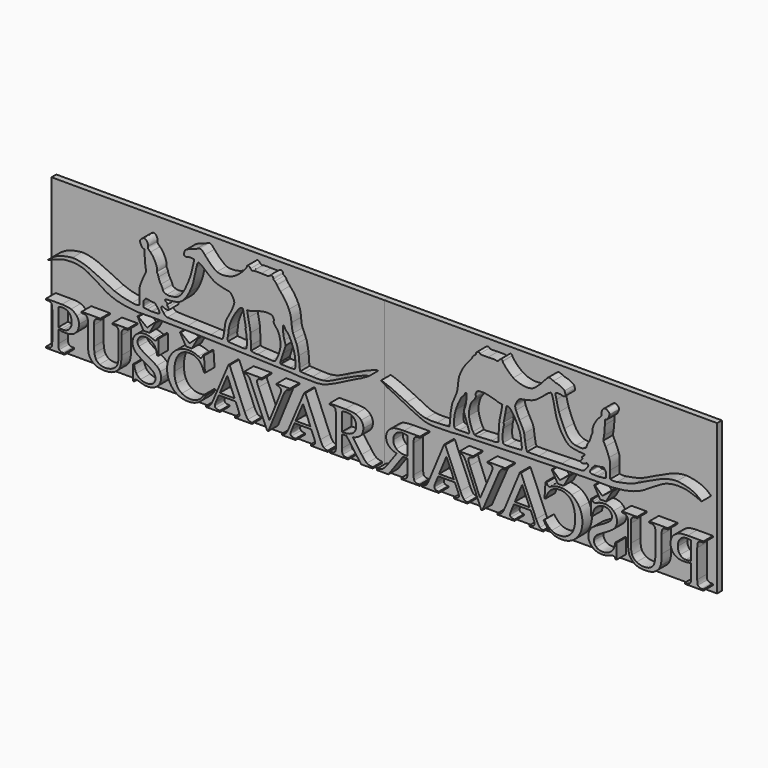
from build123d import *

# Parameters (mm, degrees)
F1_DEPTH = 2
F2_W     = 55.653892
F2_H     = 25.0897646814
F3_DEPTH = 1


# Not quite as in the source:
# - ends of sketch curves that miss each other by under 0.0002 mm in the source are joined


with BuildPart() as f1:
    # F0 (on Front) → F1 (new body)
    with BuildSketch(Plane.XZ):
        with BuildLine():
            add(Edge.make_bspline(
                [(14.906345, -1.877976), (14.32217, -1.779452), (13.148397, -1.722864), (11.136232, -1.696216)],
                knots=[0, 0, 0, 0, 1, 1, 1, 1], degree=3))
            add(Edge.make_bspline(
                [(17.93175, -1.917631), (17.120906, -1.922429), (15.472308, -1.914696), (14.906345, -1.877976)],
                knots=[0, 0, 0, 0, 1, 1, 1, 1], degree=3))
            add(Edge.make_bspline(
                [(21.221287, -0.880716), (18.995206, -1.990873), (18.702316, -1.788918), (17.93175, -1.917631)],
                knots=[0, 0, 0, 0, 1, 1, 1, 1], degree=3))
            add(Edge.make_bspline(
                [(24.850025, 0.960048), (24.039003, 0.584379), (23.127224, 0.069786), (21.221287, -0.880716)],
                knots=[0, 0, 0, 0, 1, 1, 1, 1], degree=3))
            add(Edge.make_bspline(
                [(26.655553, 1.91644), (25.579851, 1.29154), (25.170539, 1.055504), (24.850025, 0.960048)],
                knots=[0, 0, 0, 0, 1, 1, 1, 1], degree=3))
            add(Edge.make_bspline(
                [(22.267048, 0.156324), (24.465708, 1.272403), (26.336585, 2.022764), (26.655553, 1.91644)],
                knots=[0, 0, 0, 0, 1, 1, 1, 1], degree=3))
            add(Edge.make_bspline(
                [(19.081687, -1.170408), (19.8364, -1.054392), (20.090223, -0.948672), (22.267048, 0.156324)],
                knots=[0, 0, 0, 0, 1, 1, 1, 1], degree=3))
            add(Edge.make_bspline(
                [(17.243755, -1.222769), (17.960379, -1.274655), (18.504328, -1.259159), (19.081687, -1.170408)],
                knots=[0, 0, 0, 0, 1, 1, 1, 1], degree=3))
            add(Edge.make_bspline(
                [(15.753238, -1.157751), (16.121207, -1.200516), (16.683927, -1.182247), (17.243755, -1.222769)],
                knots=[0, 0, 0, 0, 1, 1, 1, 1], degree=3))
            Line((15.753238, -1.157751), (15.198408, -1.093263))
            Line((15.198408, -1.093263), (15.088607, -0.617193))
            add(Edge.make_bspline(
                [(14.94541, 1.125097), (15.075639, 0.479813), (15.009153, -0.272688), (15.088607, -0.617193)],
                knots=[0, 0, 0, 0, 1, 1, 1, 1], degree=3))
            add(Edge.make_bspline(
                [(14.582732, 2.719921), (14.739998, 2.461315), (14.74895, 2.098563), (14.94541, 1.125097)],
                knots=[0, 0, 0, 0, 1, 1, 1, 1], degree=3))
            add(Edge.make_bspline(
                [(14.328207, 3.347891), (14.44461, 3.112924), (14.481984, 2.885585), (14.582732, 2.719921)],
                knots=[0, 0, 0, 0, 1, 1, 1, 1], degree=3))
            add(Edge.make_bspline(
                [(13.999418, 4.123104), (14.095811, 3.931701), (14.222803, 3.560655), (14.328207, 3.347891)],
                knots=[0, 0, 0, 0, 1, 1, 1, 1], degree=3))
            add(Edge.make_bspline(
                [(13.727534, 5.573331), (13.790834, 4.851254), (13.884605, 4.351086), (13.999418, 4.123104)],
                knots=[0, 0, 0, 0, 1, 1, 1, 1], degree=3))
            add(Edge.make_bspline(
                [(13.308524, 7.419482), (13.576491, 6.801128), (13.647219, 6.489506), (13.727534, 5.573331)],
                knots=[0, 0, 0, 0, 1, 1, 1, 1], degree=3))
            add(Edge.make_bspline(
                [(11.873043, 9.590299), (12.525854, 8.877087), (12.963999, 8.214497), (13.308524, 7.419482)],
                knots=[0, 0, 0, 0, 1, 1, 1, 1], degree=3))
            add(Edge.make_bspline(
                [(11.312471, 10.358717), (11.397874, 10.179621), (11.650133, 9.833834), (11.873043, 9.590299)],
                knots=[0, 0, 0, 0, 1, 1, 1, 1], degree=3))
            add(Edge.make_bspline(
                [(10.93464, 10.785747), (11.057043, 10.729977), (11.227065, 10.537815), (11.312471, 10.358717)],
                knots=[0, 0, 0, 0, 1, 1, 1, 1], degree=3))
            add(Edge.make_bspline(
                [(10.712094, 11.058823), (10.712094, 10.964399), (10.81224, 10.841517), (10.93464, 10.785747)],
                knots=[0, 0, 0, 0, 1, 1, 1, 1], degree=3))
            add(Edge.make_bspline(
                [(10.041345, 11.302095), (10.278685, 11.588074), (10.712094, 11.430879), (10.712094, 11.058823)],
                knots=[0, 0, 0, 0, 1, 1, 1, 1], degree=3))
            add(Edge.make_bspline(
                [(8.698811, 11.201489), (9.752135, 11.154643), (9.930034, 11.167972), (10.041345, 11.302095)],
                knots=[0, 0, 0, 0, 1, 1, 1, 1], degree=3))
            add(Edge.make_bspline(
                [(7.316055, 11.150237), (7.429841, 11.221298), (7.879037, 11.237946), (8.698811, 11.201489)],
                knots=[0, 0, 0, 0, 1, 1, 1, 1], degree=3))
            add(Edge.make_bspline(
                [(6.894993, 11.345097), (7.105031, 11.09548), (7.175878, 11.062695), (7.316055, 11.150237)],
                knots=[0, 0, 0, 0, 1, 1, 1, 1], degree=3))
            add(Edge.make_bspline(
                [(6.253564, 11.386014), (6.324227, 11.736813), (6.579065, 11.720557), (6.894993, 11.345097)],
                knots=[0, 0, 0, 0, 1, 1, 1, 1], degree=3))
            add(Edge.make_bspline(
                [(4.478759, 9.532788), (5.163673, 9.984654), (6.186398, 11.052569), (6.253564, 11.386014)],
                knots=[0, 0, 0, 0, 1, 1, 1, 1], degree=3))
            add(Edge.make_bspline(
                [(1.271998, 9.038063), (2.051735, 8.694703), (3.561472, 8.927619), (4.478759, 9.532788)],
                knots=[0, 0, 0, 0, 1, 1, 1, 1], degree=3))
            add(Edge.make_bspline(
                [(-0.752399, 10.868156), (-0.091398, 10.050352), (0.796987, 9.247235), (1.271998, 9.038063)],
                knots=[0, 0, 0, 0, 1, 1, 1, 1], degree=3))
            add(Edge.make_bspline(
                [(-2.225738, 11.266098), (-1.473508, 11.658181), (-1.367889, 11.629654), (-0.752399, 10.868156)],
                knots=[0, 0, 0, 0, 1, 1, 1, 1], degree=3))
            add(Edge.make_bspline(
                [(-2.774897, 11.079693), (-2.669555, 11.079693), (-2.42243, 11.163575), (-2.225738, 11.266098)],
                knots=[0, 0, 0, 0, 1, 1, 1, 1], degree=3))
            add(Edge.make_bspline(
                [(-4.08105, 10.424963), (-3.987386, 10.604222), (-3.038848, 11.079693), (-2.774897, 11.079693)],
                knots=[0, 0, 0, 0, 1, 1, 1, 1], degree=3))
            add(Edge.make_bspline(
                [(-4.219618, 9.989076), (-4.185483, 10.148283), (-4.123126, 10.344431), (-4.08105, 10.424963)],
                knots=[0, 0, 0, 0, 1, 1, 1, 1], degree=3))
            add(Edge.make_bspline(
                [(-4.061568, 9.599316), (-4.246722, 9.683681), (-4.271826, 9.745583), (-4.219618, 9.989076)],
                knots=[0, 0, 0, 0, 1, 1, 1, 1], degree=3))
            add(Edge.make_bspline(
                [(-3.610077, 9.613738), (-3.778781, 9.530104), (-3.901071, 9.526198), (-4.061568, 9.599316)],
                knots=[0, 0, 0, 0, 1, 1, 1, 1], degree=3))
            add(Edge.make_bspline(
                [(-2.931005, 9.687685), (-3.179434, 9.710291), (-3.481691, 9.677384), (-3.610077, 9.613738)],
                knots=[0, 0, 0, 0, 1, 1, 1, 1], degree=3))
            add(Edge.make_bspline(
                [(-2.725248, 8.702524), (-2.519345, 9.684477), (-2.413054, 9.640532), (-2.931005, 9.687685)],
                knots=[0, 0, 0, 0, 1, 1, 1, 1], degree=3))
            add(Edge.make_bspline(
                [(-3.15726, 6.987366), (-2.958632, 7.561011), (-2.79805, 8.355337), (-2.725248, 8.702524)],
                knots=[0, 0, 0, 0, 1, 1, 1, 1], degree=3))
            add(Edge.make_bspline(
                [(-4.059426, 4.808949), (-3.614686, 5.727312), (-3.417731, 6.235111), (-3.15726, 6.987366)],
                knots=[0, 0, 0, 0, 1, 1, 1, 1], degree=3))
            add(Edge.make_bspline(
                [(-6.004577, 2.986056), (-5.607307, 3.019452), (-4.839203, 3.198762), (-4.059426, 4.808949)],
                knots=[0, 0, 0, 0, 1, 1, 1, 1], degree=3))
            add(Edge.make_bspline(
                [(-7.133794, 2.942523), (-6.823922, 2.823849), (-6.26808, 2.963916), (-6.004577, 2.986056)],
                knots=[0, 0, 0, 0, 1, 1, 1, 1], degree=3))
            add(Edge.make_bspline(
                [(-7.76966, 3.423622), (-7.718225, 3.172137), (-7.620435, 3.128897), (-7.133794, 2.942523)],
                knots=[0, 0, 0, 0, 1, 1, 1, 1], degree=3))
            add(Edge.make_bspline(
                [(-8.10803, 4.135725), (-7.954679, 3.904204), (-7.802412, 3.583758), (-7.76966, 3.423622)],
                knots=[0, 0, 0, 0, 1, 1, 1, 1], degree=3))
            add(Edge.make_bspline(
                [(-8.505055, 5.084853), (-8.440045, 4.79435), (-8.261384, 4.367243), (-8.10803, 4.135725)],
                knots=[0, 0, 0, 0, 1, 1, 1, 1], degree=3))
            add(Edge.make_bspline(
                [(-8.717103, 5.613037), (-8.665487, 5.613037), (-8.570068, 5.375352), (-8.505055, 5.084853)],
                knots=[0, 0, 0, 0, 1, 1, 1, 1], degree=3))
            add(Edge.make_bspline(
                [(-8.753904, 5.792768), (-8.785276, 5.693914), (-8.768721, 5.613037), (-8.717103, 5.613037)],
                knots=[0, 0, 0, 0, 1, 1, 1, 1], degree=3))
            add(Edge.make_bspline(
                [(-9.860368, 8.304478), (-9.203417, 7.699323), (-8.59043, 6.307826), (-8.753904, 5.792768)],
                knots=[0, 0, 0, 0, 1, 1, 1, 1], degree=3))
            add(Edge.make_bspline(
                [(-10.277738, 8.987698), (-10.318358, 8.775202), (-10.250137, 8.663509), (-9.860368, 8.304478)],
                knots=[0, 0, 0, 0, 1, 1, 1, 1], degree=3))
            add(Edge.make_bspline(
                [(-11.029922, 9.981411), (-10.634264, 10.121534), (-10.176578, 9.516885), (-10.277738, 8.987698)],
                knots=[0, 0, 0, 0, 1, 1, 1, 1], degree=3))
            add(Edge.make_bspline(
                [(-11.625832, 9.412821), (-11.625832, 9.560629), (-11.276268, 9.894165), (-11.029922, 9.981411)],
                knots=[0, 0, 0, 0, 1, 1, 1, 1], degree=3))
            add(Edge.make_bspline(
                [(-11.426944, 8.863732), (-11.536331, 9.096444), (-11.625832, 9.343532), (-11.625832, 9.412821)],
                knots=[0, 0, 0, 0, 1, 1, 1, 1], degree=3))
            add(Edge.make_bspline(
                [(-11.017363, 8.440622), (-11.174629, 8.440622), (-11.278492, 8.547917), (-11.426944, 8.863732)],
                knots=[0, 0, 0, 0, 1, 1, 1, 1], degree=3))
            add(Edge.make_bspline(
                [(-10.814299, 7.568784), (-10.806933, 8.410669), (-10.814017, 8.440622), (-11.017363, 8.440622)],
                knots=[0, 0, 0, 0, 1, 1, 1, 1], degree=3))
            add(Edge.make_bspline(
                [(-10.689455, 5.941008), (-10.762316, 6.356772), (-10.818496, 7.089271), (-10.814299, 7.568784)],
                knots=[0, 0, 0, 0, 1, 1, 1, 1], degree=3))
            Line((-10.689455, 5.941008), (-10.556977, 5.185073))
            Line((-10.556977, 5.185073), (-10.933549, 4.432964))
            add(Edge.make_bspline(
                [(-11.528657, 3.000977), (-11.408461, 3.374908), (-11.140663, 4.019303), (-10.933549, 4.432964)],
                knots=[0, 0, 0, 0, 1, 1, 1, 1], degree=3))
            add(Edge.make_bspline(
                [(-11.680447, 1.180009), (-11.741371, 2.221567), (-11.728129, 2.380402), (-11.528657, 3.000977)],
                knots=[0, 0, 0, 0, 1, 1, 1, 1], degree=3))
            add(Edge.make_bspline(
                [(-11.725561, -0.095861), (-11.644368, 0.001968), (-11.632001, 0.351755), (-11.680447, 1.180009)],
                knots=[0, 0, 0, 0, 1, 1, 1, 1], degree=3))
            add(Edge.make_bspline(
                [(-12.910174, -0.133882), (-12.705955, -0.185907), (-11.856695, -0.253869), (-11.725561, -0.095861)],
                knots=[0, 0, 0, 0, 1, 1, 1, 1], degree=3))
            add(Edge.make_bspline(
                [(-15.904108, 0.64861), (-14.299201, 0.005744), (-13.8899, 0.095759), (-12.910174, -0.133882)],
                knots=[0, 0, 0, 0, 1, 1, 1, 1], degree=3))
            add(Edge.make_bspline(
                [(-22.904303, 3.242929), (-20.452492, 3.2672), (-17.509014, 1.291476), (-15.904108, 0.64861)],
                knots=[0, 0, 0, 0, 1, 1, 1, 1], degree=3))
            add(Edge.make_bspline(
                [(-26.998339, 1.579359), (-25.865313, 2.728317), (-24.513767, 3.060715), (-22.904303, 3.242929)],
                knots=[0, 0, 0, 0, 1, 1, 1, 1], degree=3))
            add(Edge.make_bspline(
                [(-22.929805, 2.60097), (-24.746773, 2.592249), (-25.035387, 2.340363), (-26.998339, 1.579359)],
                knots=[0, 0, 0, 0, 1, 1, 1, 1], degree=3))
            add(Edge.make_bspline(
                [(-17.952161, 0.517718), (-20.188597, 1.791212), (-20.672504, 2.477729), (-22.929805, 2.60097)],
                knots=[0, 0, 0, 0, 1, 1, 1, 1], degree=3))
            add(Edge.make_bspline(
                [(-9.194343, -1.180633), (-13.817713, -1.465037), (-16.547222, -0.573734), (-17.952161, 0.517718)],
                knots=[0, 0, 0, 0, 1, 1, 1, 1], degree=3))
            add(Edge.make_bspline(
                [(-3.162159, -1.26493), (-3.716969, -1.21299), (-6.431622, -1.212044), (-9.194343, -1.180633)],
                knots=[0, 0, 0, 0, 1, 1, 1, 1], degree=3))
            add(Edge.make_bspline(
                [(1.993705, -1.411014), (-0.287212, -1.382608), (-2.607353, -1.31687), (-3.162159, -1.26493)],
                knots=[0, 0, 0, 0, 1, 1, 1, 1], degree=3))
            add(Edge.make_bspline(
                [(7.177613, -1.560089), (6.607383, -1.506504), (4.274625, -1.43942), (1.993705, -1.411014)],
                knots=[0, 0, 0, 0, 1, 1, 1, 1], degree=3))
            add(Edge.make_bspline(
                [(11.136232, -1.696216), (9.529222, -1.674937), (7.747843, -1.613678), (7.177613, -1.560089)],
                knots=[0, 0, 0, 0, 1, 1, 1, 1], degree=3))
        make_face()
        with BuildLine():
            add(Edge.make_bspline(
                [(-8.910165, -0.345128), (-8.490871, -0.342588), (-8.182475, -0.281318), (-8.373864, 0.074051)],
                knots=[0, 0, 0, 0, 1, 1, 1, 1], degree=3))
            add(Edge.make_bspline(
                [(-9.495381, -0.358754), (-9.387612, -0.349412), (-9.289241, -0.364709), (-8.910165, -0.345128)],
                knots=[0, 0, 0, 0, 1, 1, 1, 1], degree=3))
            add(Edge.make_bspline(
                [(-9.738335, -0.368462), (-9.638846, -0.372809), (-9.59257, -0.361435), (-9.495381, -0.358754)],
                knots=[0, 0, 0, 0, 1, 1, 1, 1], degree=3))
            add(Edge.make_bspline(
                [(-10.404219, -0.294599), (-10.152152, -0.315992), (-9.923366, -0.360371), (-9.738335, -0.368462)],
                knots=[0, 0, 0, 0, 1, 1, 1, 1], degree=3))
            add(Edge.make_bspline(
                [(-10.839261, -0.242123), (-10.691761, -0.281312), (-10.522207, -0.284589), (-10.404219, -0.294599)],
                knots=[0, 0, 0, 0, 1, 1, 1, 1], degree=3))
            add(Edge.make_bspline(
                [(-11.026996, 0.280505), (-11.000777, -0.125859), (-11.080697, -0.177971), (-10.839261, -0.242123)],
                knots=[0, 0, 0, 0, 1, 1, 1, 1], degree=3))
            add(Edge.make_bspline(
                [(-10.914375, 0.886837), (-10.999324, 0.787582), (-11.045656, 0.569619), (-11.026996, 0.280505)],
                knots=[0, 0, 0, 0, 1, 1, 1, 1], degree=3))
            add(Edge.make_bspline(
                [(-10.715185, 1.149182), (-10.746774, 1.059983), (-10.841429, 0.972062), (-10.914375, 0.886837)],
                knots=[0, 0, 0, 0, 1, 1, 1, 1], degree=3))
            add(Edge.make_bspline(
                [(-10.392712, 1.227538), (-10.479397, 1.236061), (-10.662466, 1.298051), (-10.715185, 1.149182)],
                knots=[0, 0, 0, 0, 1, 1, 1, 1], degree=3))
            add(Edge.make_bspline(
                [(-9.543734, 1.088922), (-9.794588, 1.088922), (-10.164671, 1.205107), (-10.392712, 1.227538)],
                knots=[0, 0, 0, 0, 1, 1, 1, 1], degree=3))
            add(Edge.make_bspline(
                [(-8.986752, 0.900417), (-9.066299, 1.049052), (-9.184099, 1.088922), (-9.543734, 1.088922)],
                knots=[0, 0, 0, 0, 1, 1, 1, 1], degree=3))
            add(Edge.make_bspline(
                [(-8.78139, 0.684514), (-8.911655, 0.723077), (-8.927756, 0.790184), (-8.986752, 0.900417)],
                knots=[0, 0, 0, 0, 1, 1, 1, 1], degree=3))
            add(Edge.make_bspline(
                [(-8.607045, 0.434798), (-8.682339, 0.537321), (-8.674041, 0.652736), (-8.78139, 0.684514)],
                knots=[0, 0, 0, 0, 1, 1, 1, 1], degree=3))
            add(Edge.make_bspline(
                [(-8.373864, 0.074051), (-8.403811, 0.147174), (-8.50376, 0.294159), (-8.607045, 0.434798)],
                knots=[0, 0, 0, 0, 1, 1, 1, 1], degree=3))
        make_face(mode=Mode.SUBTRACT)
        with BuildLine():
            add(Edge.make_bspline(
                [(-7.048802, 1.502837), (-7.127644, 1.407839), (-6.992671, 1.331672), (-6.912331, 1.181793)],
                knots=[0, 0, 0, 0, 1, 1, 1, 1], degree=3))
            add(Edge.make_bspline(
                [(-7.01613, 2.215528), (-8.157323, 2.174605), (-6.659226, 1.665838), (-7.048802, 1.502837)],
                knots=[0, 0, 0, 0, 1, 1, 1, 1], degree=3))
            add(Edge.make_bspline(
                [(-5.578315, 2.386771), (-5.898216, 2.288126), (-6.814231, 2.205943), (-7.01613, 2.215528)],
                knots=[0, 0, 0, 0, 1, 1, 1, 1], degree=3))
            add(Edge.make_bspline(
                [(-4.531857, 2.871073), (-4.817808, 2.612456), (-5.229875, 2.43191), (-5.578315, 2.386771)],
                knots=[0, 0, 0, 0, 1, 1, 1, 1], degree=3))
            add(Edge.make_bspline(
                [(-3.354824, 4.508436), (-3.671204, 3.862607), (-4.280098, 3.049649), (-4.531857, 2.871073)],
                knots=[0, 0, 0, 0, 1, 1, 1, 1], degree=3))
            add(Edge.make_bspline(
                [(-2.175694, 8.560992), (-2.56428, 6.342971), (-2.855096, 5.528526), (-3.354824, 4.508436)],
                knots=[0, 0, 0, 0, 1, 1, 1, 1], degree=3))
            add(Edge.make_bspline(
                [(-1.750597, 9.378886), (-1.916109, 9.383035), (-1.998193, 9.290254), (-2.175694, 8.560992)],
                knots=[0, 0, 0, 0, 1, 1, 1, 1], degree=3))
            add(Edge.make_bspline(
                [(-1.01849, 8.928364), (-1.281574, 9.170691), (-1.530667, 9.303115), (-1.750597, 9.378886)],
                knots=[0, 0, 0, 0, 1, 1, 1, 1], degree=3))
            add(Edge.make_bspline(
                [(1.060771, 7.356657), (0.581654, 7.56871), (-0.109819, 8.091391), (-1.01849, 8.928364)],
                knots=[0, 0, 0, 0, 1, 1, 1, 1], degree=3))
            add(Edge.make_bspline(
                [(3.218205, 6.838342), (2.839519, 6.838342), (1.510394, 7.157659), (1.060771, 7.356657)],
                knots=[0, 0, 0, 0, 1, 1, 1, 1], degree=3))
            add(Edge.make_bspline(
                [(4.060283, 5.880124), (3.873068, 6.370341), (3.461791, 6.838342), (3.218205, 6.838342)],
                knots=[0, 0, 0, 0, 1, 1, 1, 1], degree=3))
            add(Edge.make_bspline(
                [(4.033076, 4.899018), (4.214246, 5.435282), (4.215321, 5.474133), (4.060283, 5.880124)],
                knots=[0, 0, 0, 0, 1, 1, 1, 1], degree=3))
            add(Edge.make_bspline(
                [(3.448512, 3.633745), (3.666272, 4.02254), (3.929329, 4.591912), (4.033076, 4.899018)],
                knots=[0, 0, 0, 0, 1, 1, 1, 1], degree=3))
            add(Edge.make_bspline(
                [(2.663192, 1.913468), (2.757802, 2.28428), (2.756721, 2.398614), (3.448512, 3.633745)],
                knots=[0, 0, 0, 0, 1, 1, 1, 1], degree=3))
            add(Edge.make_bspline(
                [(2.512378, 0.792608), (2.600587, 1.204351), (2.582412, 1.596865), (2.663192, 1.913468)],
                knots=[0, 0, 0, 0, 1, 1, 1, 1], degree=3))
            add(Edge.make_bspline(
                [(2.327497, -0.227682), (2.400339, -0.041381), (2.435526, 0.43387), (2.512378, 0.792608)],
                knots=[0, 0, 0, 0, 1, 1, 1, 1], degree=3))
            Line((2.327497, -0.227682), (2.181902, -0.600062))
            add(Edge.make_bspline(
                [(0.232009, -0.576553), (0.872563, -0.617182), (1.590502, -0.61016), (2.181902, -0.600062)],
                knots=[0, 0, 0, 0, 1, 1, 1, 1], degree=3))
            add(Edge.make_bspline(
                [(-3.590776, -0.472679), (-2.393361, -0.51865), (-0.800696, -0.520315), (0.232009, -0.576553)],
                knots=[0, 0, 0, 0, 1, 1, 1, 1], degree=3))
            add(Edge.make_bspline(
                [(-7.041067, -0.368403), (-6.859287, -0.402507), (-5.306659, -0.449429), (-3.590776, -0.472679)],
                knots=[0, 0, 0, 0, 1, 1, 1, 1], degree=3))
            add(Edge.make_bspline(
                [(-7.632221, 0.08488), (-7.435851, -0.209899), (-7.290057, -0.321693), (-7.041067, -0.368403)],
                knots=[0, 0, 0, 0, 1, 1, 1, 1], degree=3))
            add(Edge.make_bspline(
                [(-8.025351, 0.604434), (-7.940803, 0.419496), (-7.781937, 0.282607), (-7.632221, 0.08488)],
                knots=[0, 0, 0, 0, 1, 1, 1, 1], degree=3))
            add(Edge.make_bspline(
                [(-8.01615, 0.874371), (-8.063264, 0.771642), (-8.052681, 0.682654), (-8.025351, 0.604434)],
                knots=[0, 0, 0, 0, 1, 1, 1, 1], degree=3))
            add(Edge.make_bspline(
                [(-7.581759, 0.873524), (-7.839657, 1.025868), (-7.864676, 1.025919), (-8.01615, 0.874371)],
                knots=[0, 0, 0, 0, 1, 1, 1, 1], degree=3))
            add(Edge.make_bspline(
                [(-6.912331, 1.181793), (-6.43918, 0.721799), (-7.058514, 0.564434), (-7.581759, 0.873524)],
                knots=[0, 0, 0, 0, 1, 1, 1, 1], degree=3))
        make_face(mode=Mode.SUBTRACT)
        with BuildLine():
            add(Edge.make_bspline(
                [(6.184643, -0.613849), (6.328788, -0.34451), (6.305863, 1.196601), (6.152122, 1.572216)],
                knots=[0, 0, 0, 0, 1, 1, 1, 1], degree=3))
            add(Edge.make_bspline(
                [(5.501306, -0.781379), (5.992971, -0.793769), (6.102745, -0.766873), (6.184643, -0.613849)],
                knots=[0, 0, 0, 0, 1, 1, 1, 1], degree=3))
            add(Edge.make_bspline(
                [(3.121473, -0.611176), (3.164935, -0.656425), (4.563654, -0.757717), (5.501306, -0.781379)],
                knots=[0, 0, 0, 0, 1, 1, 1, 1], degree=3))
            add(Edge.make_bspline(
                [(3.08674, 0.094678), (3.016108, -0.268195), (3.099525, -0.588342), (3.121473, -0.611176)],
                knots=[0, 0, 0, 0, 1, 1, 1, 1], degree=3))
            add(Edge.make_bspline(
                [(3.223189, 1.063934), (3.221213, 0.891205), (3.157369, 0.457551), (3.08674, 0.094678)],
                knots=[0, 0, 0, 0, 1, 1, 1, 1], degree=3))
            add(Edge.make_bspline(
                [(4.238692, 3.760612), (3.644372, 2.802936), (3.229257, 1.613852), (3.223189, 1.063934)],
                knots=[0, 0, 0, 0, 1, 1, 1, 1], degree=3))
            add(Edge.make_bspline(
                [(5.440293, 5.04752), (5.14241, 5.04752), (4.829064, 4.71193), (4.238692, 3.760612)],
                knots=[0, 0, 0, 0, 1, 1, 1, 1], degree=3))
            add(Edge.make_bspline(
                [(5.860931, 3.680854), (5.668032, 4.980261), (5.647328, 5.04752), (5.440293, 5.04752)],
                knots=[0, 0, 0, 0, 1, 1, 1, 1], degree=3))
            add(Edge.make_bspline(
                [(6.088227, 2.470529), (6.070475, 2.563722), (5.945584, 3.110624), (5.860931, 3.680854)],
                knots=[0, 0, 0, 0, 1, 1, 1, 1], degree=3))
            add(Edge.make_bspline(
                [(6.065339, 2.218417), (6.111804, 2.37303), (6.105979, 2.377334), (6.088227, 2.470529)],
                knots=[0, 0, 0, 0, 1, 1, 1, 1], degree=3))
            add(Edge.make_bspline(
                [(6.152122, 1.572216), (6.02902, 2.126563), (6.0532, 2.178031), (6.065339, 2.218417)],
                knots=[0, 0, 0, 0, 1, 1, 1, 1], degree=3))
        make_face(mode=Mode.SUBTRACT)
        with BuildLine():
            add(Edge.make_bspline(
                [(10.972119, -0.970234), (11.068069, -0.868905), (11.124229, -0.728688), (11.217681, -0.588627)],
                knots=[0, 0, 0, 0, 1, 1, 1, 1], degree=3))
            add(Edge.make_bspline(
                [(10.441141, -1.02308), (10.61234, -1.048169), (10.813135, -1.018564), (10.972119, -0.970234)],
                knots=[0, 0, 0, 0, 1, 1, 1, 1], degree=3))
            add(Edge.make_bspline(
                [(8.089973, -0.896675), (9.030035, -0.891257), (10.360984, -1.011331), (10.441141, -1.02308)],
                knots=[0, 0, 0, 0, 1, 1, 1, 1], degree=3))
            add(Edge.make_bspline(
                [(7.32374, -0.854751), (7.497097, -0.911963), (7.710503, -0.898868), (8.089973, -0.896675)],
                knots=[0, 0, 0, 0, 1, 1, 1, 1], degree=3))
            Line((7.32374, -0.854751), (6.95689, -0.750727))
            Line((6.95689, -0.750727), (6.977267, 0.080327))
            add(Edge.make_bspline(
                [(6.849149, 1.838394), (6.842037, 1.268164), (6.987723, 0.506474), (6.977267, 0.080327)],
                knots=[0, 0, 0, 0, 1, 1, 1, 1], degree=3))
            add(Edge.make_bspline(
                [(6.496809, 3.963612), (6.615602, 3.295945), (6.857469, 2.506058), (6.849149, 1.838394)],
                knots=[0, 0, 0, 0, 1, 1, 1, 1], degree=3))
            add(Edge.make_bspline(
                [(6.32084, 5.013676), (6.316155, 5.006367), (6.395353, 4.533842), (6.496809, 3.963612)],
                knots=[0, 0, 0, 0, 1, 1, 1, 1], degree=3))
            add(Edge.make_bspline(
                [(6.708351, 5.069511), (6.499893, 5.046115), (6.325514, 5.02098), (6.32084, 5.013676)],
                knots=[0, 0, 0, 0, 1, 1, 1, 1], degree=3))
            add(Edge.make_bspline(
                [(7.320994, 5.23767), (7.192498, 5.168585), (6.916809, 5.092913), (6.708351, 5.069511)],
                knots=[0, 0, 0, 0, 1, 1, 1, 1], degree=3))
            add(Edge.make_bspline(
                [(7.931635, 5.445341), (7.724278, 5.400208), (7.449492, 5.306758), (7.320994, 5.23767)],
                knots=[0, 0, 0, 0, 1, 1, 1, 1], degree=3))
            add(Edge.make_bspline(
                [(8.685659, 5.624783), (8.478302, 5.571223), (8.138992, 5.490474), (7.931635, 5.445341)],
                knots=[0, 0, 0, 0, 1, 1, 1, 1], degree=3))
            add(Edge.make_bspline(
                [(10.391868, 5.656584), (10.064219, 5.787191), (9.25609, 5.772129), (8.685659, 5.624783)],
                knots=[0, 0, 0, 0, 1, 1, 1, 1], degree=3))
            add(Edge.make_bspline(
                [(10.747857, 4.816265), (10.866077, 5.124338), (10.691133, 5.537292), (10.391868, 5.656584)],
                knots=[0, 0, 0, 0, 1, 1, 1, 1], degree=3))
            add(Edge.make_bspline(
                [(11.346608, 3.810075), (10.947227, 4.245696), (10.692911, 4.673073), (10.747857, 4.816265)],
                knots=[0, 0, 0, 0, 1, 1, 1, 1], degree=3))
            add(Edge.make_bspline(
                [(11.900563, 1.529146), (11.972182, 2.230514), (11.675756, 3.45106), (11.346608, 3.810075)],
                knots=[0, 0, 0, 0, 1, 1, 1, 1], degree=3))
            add(Edge.make_bspline(
                [(11.217681, -0.588627), (11.478573, -0.197625), (11.838087, 0.917311), (11.900563, 1.529146)],
                knots=[0, 0, 0, 0, 1, 1, 1, 1], degree=3))
        make_face(mode=Mode.SUBTRACT)
        with BuildLine():
            add(Edge.make_bspline(
                [(14.334526, -0.937535), (14.482323, -0.389691), (14.380808, 0.80618), (14.112513, 1.677778)],
                knots=[0, 0, 0, 0, 1, 1, 1, 1], degree=3))
            add(Edge.make_bspline(
                [(13.511101, -1.127155), (14.203386, -1.126026), (14.288956, -1.106468), (14.334526, -0.937535)],
                knots=[0, 0, 0, 0, 1, 1, 1, 1], degree=3))
            add(Edge.make_bspline(
                [(12.093239, -1.099074), (12.447919, -1.119591), (13.086187, -1.127759), (13.511101, -1.127155)],
                knots=[0, 0, 0, 0, 1, 1, 1, 1], degree=3))
            Line((12.093239, -1.099074), (11.904525, -1.088152))
            Line((11.904525, -1.088152), (11.839699, -0.824339))
            add(Edge.make_bspline(
                [(12.335636, 0.628942), (12.095635, -0.091221), (11.874361, -0.684263), (11.839699, -0.824339)],
                knots=[0, 0, 0, 0, 1, 1, 1, 1], degree=3))
            Line((12.335636, 0.628942), (12.768554, 1.927988))
            Line((12.768554, 1.927988), (12.541475, 2.643069))
            add(Edge.make_bspline(
                [(12.404222, 4.764762), (12.218469, 4.764762), (12.308199, 3.377654), (12.541475, 2.643069)],
                knots=[0, 0, 0, 0, 1, 1, 1, 1], degree=3))
            add(Edge.make_bspline(
                [(12.65214, 4.431615), (12.565193, 4.614845), (12.453631, 4.764762), (12.404222, 4.764762)],
                knots=[0, 0, 0, 0, 1, 1, 1, 1], degree=3))
            add(Edge.make_bspline(
                [(12.987113, 4.003806), (12.889828, 4.055873), (12.73909, 4.248388), (12.65214, 4.431615)],
                knots=[0, 0, 0, 0, 1, 1, 1, 1], degree=3))
            add(Edge.make_bspline(
                [(14.112513, 1.677778), (13.788308, 2.731009), (13.237266, 3.869928), (12.987113, 4.003806)],
                knots=[0, 0, 0, 0, 1, 1, 1, 1], degree=3))
        make_face(mode=Mode.SUBTRACT)
    extrude(amount=F1_DEPTH)



with BuildPart() as f1b:
    # F0 (on Front) → F1, piece 2 (new body)
    with BuildSketch(Plane.XZ):
        with BuildLine():
            add(Edge.make_bspline(
                [(-25.247666, -10.180231), (-25.247668, -10.637627), (-25.197973, -10.921713), (-25.098579, -11.032487)],
                knots=[0, 0, 0, 0, 1, 1, 1, 1], degree=3))
            Line((-25.247666, -10.180231), (-25.247666, -8.062994))
            add(Edge.make_bspline(
                [(-24.598073, -8.175554), (-24.800408, -8.150551), (-25.016939, -8.113023), (-25.247666, -8.062994)],
                knots=[0, 0, 0, 0, 1, 1, 1, 1], degree=3))
            add(Edge.make_bspline(
                [(-24.033673, -8.213076), (-24.207611, -8.213079), (-24.395744, -8.20056), (-24.598073, -8.175554)],
                knots=[0, 0, 0, 0, 1, 1, 1, 1], degree=3))
            add(Edge.make_bspline(
                [(-22.38573, -7.655627), (-22.774426, -8.027261), (-23.32374, -8.213079), (-24.033673, -8.213076)],
                knots=[0, 0, 0, 0, 1, 1, 1, 1], degree=3))
            add(Edge.make_bspline(
                [(-21.802694, -6.208399), (-21.8027, -6.801586), (-21.997045, -7.283995), (-22.38573, -7.655627)],
                knots=[0, 0, 0, 0, 1, 1, 1, 1], degree=3))
            add(Edge.make_bspline(
                [(-22.18606, -5.077417), (-21.930488, -5.395457), (-21.8027, -5.772449), (-21.802694, -6.208399)],
                knots=[0, 0, 0, 0, 1, 1, 1, 1], degree=3))
            add(Edge.make_bspline(
                [(-23.128502, -4.399365), (-22.75579, -4.533375), (-22.441643, -4.759393), (-22.18606, -5.077417)],
                knots=[0, 0, 0, 0, 1, 1, 1, 1], degree=3))
            add(Edge.make_bspline(
                [(-24.656643, -4.198362), (-24.010603, -4.198368), (-23.501224, -4.26537), (-23.128502, -4.399365)],
                knots=[0, 0, 0, 0, 1, 1, 1, 1], degree=3))
            Line((-24.656643, -4.198362), (-27.302936, -4.198362))
            Line((-27.302936, -4.198362), (-27.302936, -4.396687))
            Line((-27.302936, -4.396687), (-27.031384, -4.396687))
            add(Edge.make_bspline(
                [(-26.413739, -4.632531), (-26.552177, -4.475307), (-26.758059, -4.396692), (-27.031384, -4.396687)],
                knots=[0, 0, 0, 0, 1, 1, 1, 1], degree=3))
            add(Edge.make_bspline(
                [(-26.269976, -5.484787), (-26.269977, -5.027396), (-26.317898, -4.743313), (-26.413739, -4.632531)],
                knots=[0, 0, 0, 0, 1, 1, 1, 1], degree=3))
            Line((-26.269976, -5.484787), (-26.269976, -10.180231))
            add(Edge.make_bspline(
                [(-26.376467, -10.968166), (-26.305474, -10.85739), (-26.269977, -10.594748), (-26.269976, -10.180231)],
                knots=[0, 0, 0, 0, 1, 1, 1, 1], degree=3))
            add(Edge.make_bspline(
                [(-27.031384, -11.268331), (-26.726112, -11.268331), (-26.507806, -11.168278), (-26.376467, -10.968166)],
                knots=[0, 0, 0, 0, 1, 1, 1, 1], degree=3))
            Line((-27.031384, -11.268331), (-27.302936, -11.268331))
            Line((-27.302936, -11.268331), (-27.302936, -11.466655))
            Line((-27.302936, -11.466655), (-24.209382, -11.466655))
            Line((-24.209382, -11.466655), (-24.209382, -11.268331))
            Line((-24.209382, -11.268331), (-24.486258, -11.268331))
            add(Edge.make_bspline(
                [(-25.098579, -11.032487), (-24.963694, -11.189716), (-24.759587, -11.268331), (-24.486258, -11.268331)],
                knots=[0, 0, 0, 0, 1, 1, 1, 1], degree=3))
        make_face()
        with BuildLine():
            add(Edge.make_bspline(
                [(-25.247666, -7.757466), (-25.059535, -7.793204), (-24.8927, -7.820006), (-24.74716, -7.837868)],
                knots=[0, 0, 0, 0, 1, 1, 1, 1], degree=3))
            Line((-25.247666, -7.757466), (-25.247666, -4.734384))
            add(Edge.make_bspline(
                [(-24.550152, -4.632545), (-24.731189, -4.63255), (-24.963694, -4.666499), (-25.247666, -4.734384)],
                knots=[0, 0, 0, 0, 1, 1, 1, 1], degree=3))
            add(Edge.make_bspline(
                [(-23.751473, -4.833548), (-23.985756, -4.699552), (-24.251982, -4.63255), (-24.550152, -4.632545)],
                knots=[0, 0, 0, 0, 1, 1, 1, 1], degree=3))
            add(Edge.make_bspline(
                [(-23.20837, -5.43924), (-23.336163, -5.169453), (-23.517197, -4.967555), (-23.751473, -4.833548)],
                knots=[0, 0, 0, 0, 1, 1, 1, 1], degree=3))
            add(Edge.make_bspline(
                [(-23.016687, -6.315616), (-23.016692, -6.00116), (-23.080586, -5.709035), (-23.20837, -5.43924)],
                knots=[0, 0, 0, 0, 1, 1, 1, 1], degree=3))
            add(Edge.make_bspline(
                [(-23.418689, -7.433196), (-23.150692, -7.145542), (-23.016692, -6.773015), (-23.016687, -6.315616)],
                knots=[0, 0, 0, 0, 1, 1, 1, 1], degree=3))
            add(Edge.make_bspline(
                [(-24.374443, -7.864683), (-24.005279, -7.864686), (-23.686695, -7.720859), (-23.418689, -7.433196)],
                knots=[0, 0, 0, 0, 1, 1, 1, 1], degree=3))
            add(Edge.make_bspline(
                [(-24.74716, -7.837868), (-24.601626, -7.855735), (-24.477387, -7.864683), (-24.374443, -7.864683)],
                knots=[0, 0, 0, 0, 1, 1, 1, 1], degree=3))
        make_face(mode=Mode.SUBTRACT)
    extrude(amount=F1_DEPTH)


with BuildPart() as f1c:
    # F0 (on Front) → F1, piece 3 (new body)
    with BuildSketch(Plane.XZ):
        with BuildLine():
            add(Edge.make_bspline(
                [(-13.92771, -4.396687), (-14.211692, -4.396692), (-14.429999, -4.516402), (-14.582627, -4.755811)],
                knots=[0, 0, 0, 0, 1, 1, 1, 1], degree=3))
            Line((-13.92771, -4.396687), (-13.656161, -4.396687))
            Line((-13.656161, -4.396687), (-13.656161, -4.198362))
            Line((-13.656161, -4.198362), (-16.211935, -4.198362))
            Line((-16.211935, -4.198362), (-16.211935, -4.396687))
            Line((-16.211935, -4.396687), (-15.940384, -4.396687))
            add(Edge.make_bspline(
                [(-15.322738, -4.632531), (-15.461182, -4.475307), (-15.667064, -4.396692), (-15.940384, -4.396687)],
                knots=[0, 0, 0, 0, 1, 1, 1, 1], degree=3))
            add(Edge.make_bspline(
                [(-15.173651, -5.484787), (-15.173658, -5.03097), (-15.223353, -4.746886), (-15.322738, -4.632531)],
                knots=[0, 0, 0, 0, 1, 1, 1, 1], degree=3))
            Line((-15.173651, -5.484787), (-15.173651, -8.427479))
            add(Edge.make_bspline(
                [(-15.378646, -10.070349), (-15.241989, -9.74696), (-15.173658, -9.199336), (-15.173651, -8.427479)],
                knots=[0, 0, 0, 0, 1, 1, 1, 1], degree=3))
            add(Edge.make_bspline(
                [(-16.142716, -10.866324), (-15.770005, -10.659068), (-15.515315, -10.393744), (-15.378646, -10.070349)],
                knots=[0, 0, 0, 0, 1, 1, 1, 1], degree=3))
            add(Edge.make_bspline(
                [(-17.409955, -11.177209), (-16.937851, -11.177209), (-16.515438, -11.073582), (-16.142716, -10.866324)],
                knots=[0, 0, 0, 0, 1, 1, 1, 1], degree=3))
            add(Edge.make_bspline(
                [(-18.34441, -10.978887), (-18.090611, -11.111102), (-17.779126, -11.177209), (-17.409955, -11.177209)],
                knots=[0, 0, 0, 0, 1, 1, 1, 1], degree=3))
            add(Edge.make_bspline(
                [(-18.927446, -10.475038), (-18.792561, -10.678723), (-18.598216, -10.846672), (-18.34441, -10.978887)],
                knots=[0, 0, 0, 0, 1, 1, 1, 1], degree=3))
            add(Edge.make_bspline(
                [(-19.206984, -9.622781), (-19.155516, -9.987269), (-19.062337, -10.271355), (-18.927446, -10.475038)],
                knots=[0, 0, 0, 0, 1, 1, 1, 1], degree=3))
            add(Edge.make_bspline(
                [(-19.28419, -8.652605), (-19.284192, -8.934904), (-19.258455, -9.258297), (-19.206984, -9.622781)],
                knots=[0, 0, 0, 0, 1, 1, 1, 1], degree=3))
            Line((-19.28419, -8.652605), (-19.28419, -5.484787))
            add(Edge.make_bspline(
                [(-19.151077, -4.68077), (-19.239821, -4.80942), (-19.284192, -5.077425), (-19.28419, -5.484787)],
                knots=[0, 0, 0, 0, 1, 1, 1, 1], degree=3))
            add(Edge.make_bspline(
                [(-18.512133, -4.396687), (-18.810309, -4.396692), (-19.02329, -4.491388), (-19.151077, -4.68077)],
                knots=[0, 0, 0, 0, 1, 1, 1, 1], degree=3))
            Line((-18.512133, -4.396687), (-18.235257, -4.396687))
            Line((-18.235257, -4.396687), (-18.235257, -4.198362))
            Line((-18.235257, -4.198362), (-21.355433, -4.198362))
            Line((-21.355433, -4.198362), (-21.355433, -4.396687))
            Line((-21.355433, -4.396687), (-21.083882, -4.396687))
            add(Edge.make_bspline(
                [(-20.490196, -4.605729), (-20.612661, -4.466373), (-20.810557, -4.396692), (-21.083882, -4.396687)],
                knots=[0, 0, 0, 0, 1, 1, 1, 1], degree=3))
            add(Edge.make_bspline(
                [(-20.3065, -5.484787), (-20.306501, -5.038117), (-20.367733, -4.745099), (-20.490196, -4.605729)],
                knots=[0, 0, 0, 0, 1, 1, 1, 1], degree=3))
            Line((-20.3065, -5.484787), (-20.3065, -8.325639))
            add(Edge.make_bspline(
                [(-20.136115, -10.11591), (-20.249706, -9.797878), (-20.306501, -9.201123), (-20.3065, -8.325639)],
                knots=[0, 0, 0, 0, 1, 1, 1, 1], degree=3))
            add(Edge.make_bspline(
                [(-19.268217, -11.225451), (-19.676432, -10.950299), (-19.965732, -10.580454), (-20.136115, -10.11591)],
                knots=[0, 0, 0, 0, 1, 1, 1, 1], degree=3))
            add(Edge.make_bspline(
                [(-17.473849, -11.638179), (-18.261883, -11.638179), (-18.860005, -11.500604), (-19.268217, -11.225451)],
                knots=[0, 0, 0, 0, 1, 1, 1, 1], degree=3))
            add(Edge.make_bspline(
                [(-15.756688, -11.206692), (-16.177331, -11.494349), (-16.749717, -11.638179), (-17.473849, -11.638179)],
                knots=[0, 0, 0, 0, 1, 1, 1, 1], degree=3))
            add(Edge.make_bspline(
                [(-14.910087, -10.172192), (-15.053856, -10.574199), (-15.336056, -10.919032), (-15.756688, -11.206692)],
                knots=[0, 0, 0, 0, 1, 1, 1, 1], degree=3))
            add(Edge.make_bspline(
                [(-14.694443, -8.475721), (-14.694449, -9.204697), (-14.766331, -9.770185), (-14.910087, -10.172192)],
                knots=[0, 0, 0, 0, 1, 1, 1, 1], degree=3))
            Line((-14.694443, -8.475721), (-14.694443, -5.527666))
            add(Edge.make_bspline(
                [(-14.582627, -4.755811), (-14.657179, -4.866593), (-14.694449, -5.123878), (-14.694443, -5.527666)],
                knots=[0, 0, 0, 0, 1, 1, 1, 1], degree=3))
        make_face()
    extrude(amount=F1_DEPTH)


with BuildPart() as f1d:
    # F0 (on Front) → F1, piece 4 (new body)
    with BuildSketch(Plane.XZ):
        with BuildLine():
            add(Edge.make_bspline(
                [(-8.730968, -6.546085), (-8.794867, -6.06368), (-8.909344, -5.679541), (-9.074399, -5.393665)],
                knots=[0, 0, 0, 0, 1, 1, 1, 1], degree=3))
            Line((-8.730968, -6.546085), (-8.533959, -6.546085))
            Line((-8.533959, -6.546085), (-8.533959, -4.032199))
            Line((-8.533959, -4.032199), (-8.730968, -4.032199))
            add(Edge.make_bspline(
                [(-8.872068, -4.367204), (-8.813502, -4.311826), (-8.766469, -4.200154), (-8.730968, -4.032199)],
                knots=[0, 0, 0, 0, 1, 1, 1, 1], degree=3))
            add(Edge.make_bspline(
                [(-9.098359, -4.450287), (-9.006072, -4.450292), (-8.930643, -4.422593), (-8.872068, -4.367204)],
                knots=[0, 0, 0, 0, 1, 1, 1, 1], degree=3))
            add(Edge.make_bspline(
                [(-9.518997, -4.316283), (-9.320219, -4.405626), (-9.180007, -4.450292), (-9.098359, -4.450287)],
                knots=[0, 0, 0, 0, 1, 1, 1, 1], degree=3))
            add(Edge.make_bspline(
                [(-10.738317, -4.032199), (-10.354952, -4.032208), (-9.948513, -4.1269), (-9.518997, -4.316283)],
                knots=[0, 0, 0, 0, 1, 1, 1, 1], degree=3))
            add(Edge.make_bspline(
                [(-12.255807, -4.59769), (-11.858245, -4.220704), (-11.352414, -4.032208), (-10.738317, -4.032199)],
                knots=[0, 0, 0, 0, 1, 1, 1, 1], degree=3))
            add(Edge.make_bspline(
                [(-12.852155, -5.945754), (-12.852155, -5.424043), (-12.653374, -4.974688), (-12.255807, -4.59769)],
                knots=[0, 0, 0, 0, 1, 1, 1, 1], degree=3))
            add(Edge.make_bspline(
                [(-12.649824, -6.771209), (-12.784711, -6.521076), (-12.852155, -6.245924), (-12.852155, -5.945754)],
                knots=[0, 0, 0, 0, 1, 1, 1, 1], degree=3))
            add(Edge.make_bspline(
                [(-12.056137, -7.457302), (-12.317042, -7.250049), (-12.514937, -7.021352), (-12.649824, -6.771209)],
                knots=[0, 0, 0, 0, 1, 1, 1, 1], degree=3))
            add(Edge.make_bspline(
                [(-10.738317, -8.290796), (-11.355964, -7.942394), (-11.795237, -7.664563), (-12.056137, -7.457302)],
                knots=[0, 0, 0, 0, 1, 1, 1, 1], degree=3))
            add(Edge.make_bspline(
                [(-9.60419, -8.97421), (-9.742632, -8.86701), (-10.120673, -8.639205), (-10.738317, -8.290796)],
                knots=[0, 0, 0, 0, 1, 1, 1, 1], degree=3))
            add(Edge.make_bspline(
                [(-9.148942, -9.48342), (-9.246565, -9.301179), (-9.398312, -9.131442), (-9.60419, -8.97421)],
                knots=[0, 0, 0, 0, 1, 1, 1, 1], degree=3))
            add(Edge.make_bspline(
                [(-9.00252, -10.024788), (-9.002523, -9.846121), (-9.051331, -9.665664), (-9.148942, -9.48342)],
                knots=[0, 0, 0, 0, 1, 1, 1, 1], degree=3))
            add(Edge.make_bspline(
                [(-9.388546, -10.860964), (-9.131199, -10.62512), (-9.002523, -10.346397), (-9.00252, -10.024788)],
                knots=[0, 0, 0, 0, 1, 1, 1, 1], degree=3))
            add(Edge.make_bspline(
                [(-10.440141, -11.214731), (-9.996435, -11.214731), (-9.645904, -11.096807), (-9.388546, -10.860964)],
                knots=[0, 0, 0, 0, 1, 1, 1, 1], degree=3))
            add(Edge.make_bspline(
                [(-11.497062, -10.957446), (-11.175818, -11.128969), (-10.823512, -11.214731), (-10.440141, -11.214731)],
                knots=[0, 0, 0, 0, 1, 1, 1, 1], degree=3))
            add(Edge.make_bspline(
                [(-12.213212, -10.311553), (-12.057026, -10.570625), (-11.818311, -10.785923), (-11.497062, -10.957446)],
                knots=[0, 0, 0, 0, 1, 1, 1, 1], degree=3))
            add(Edge.make_bspline(
                [(-12.585927, -9.140373), (-12.493638, -9.66209), (-12.369398, -10.052484), (-12.213212, -10.311553)],
                knots=[0, 0, 0, 0, 1, 1, 1, 1], degree=3))
            Line((-12.585927, -9.140373), (-12.782936, -9.140373))
            Line((-12.782936, -9.140373), (-12.782936, -11.632818))
            Line((-12.782936, -11.632818), (-12.585927, -11.632818))
            add(Edge.make_bspline(
                [(-12.47145, -11.300492), (-12.522923, -11.354092), (-12.561082, -11.464869), (-12.585927, -11.632818)],
                knots=[0, 0, 0, 0, 1, 1, 1, 1], degree=3))
            add(Edge.make_bspline(
                [(-12.261131, -11.220091), (-12.349876, -11.220091), (-12.419981, -11.246907), (-12.47145, -11.300492)],
                knots=[0, 0, 0, 0, 1, 1, 1, 1], degree=3))
            add(Edge.make_bspline(
                [(-11.603553, -11.388933), (-11.949648, -11.276373), (-12.168842, -11.220091), (-12.261131, -11.220091)],
                knots=[0, 0, 0, 0, 1, 1, 1, 1], degree=3))
            add(Edge.make_bspline(
                [(-10.919349, -11.584579), (-11.029393, -11.566711), (-11.257461, -11.501496), (-11.603553, -11.388933)],
                knots=[0, 0, 0, 0, 1, 1, 1, 1], degree=3))
            add(Edge.make_bspline(
                [(-10.328328, -11.632818), (-10.537761, -11.632818), (-10.73477, -11.616735), (-10.919349, -11.584579)],
                knots=[0, 0, 0, 0, 1, 1, 1, 1], degree=3))
            add(Edge.make_bspline(
                [(-8.691034, -11.035168), (-9.115225, -11.433602), (-9.660989, -11.632818), (-10.328328, -11.632818)],
                knots=[0, 0, 0, 0, 1, 1, 1, 1], degree=3))
            add(Edge.make_bspline(
                [(-8.054752, -9.612061), (-8.054757, -10.162366), (-8.266851, -10.636735), (-8.691034, -11.035168)],
                knots=[0, 0, 0, 0, 1, 1, 1, 1], degree=3))
            add(Edge.make_bspline(
                [(-8.254422, -8.781246), (-8.121315, -9.045681), (-8.054757, -9.322617), (-8.054752, -9.612061)],
                knots=[0, 0, 0, 0, 1, 1, 1, 1], degree=3))
            add(Edge.make_bspline(
                [(-8.824146, -8.092474), (-8.577448, -8.287228), (-8.387539, -8.516817), (-8.254422, -8.781246)],
                knots=[0, 0, 0, 0, 1, 1, 1, 1], degree=3))
            add(Edge.make_bspline(
                [(-10.205863, -7.253617), (-9.531427, -7.618107), (-9.070855, -7.897725), (-8.824146, -8.092474)],
                knots=[0, 0, 0, 0, 1, 1, 1, 1], degree=3))
            add(Edge.make_bspline(
                [(-11.776599, -6.181598), (-11.55652, -6.449609), (-11.032943, -6.806947), (-10.205863, -7.253617)],
                knots=[0, 0, 0, 0, 1, 1, 1, 1], degree=3))
            add(Edge.make_bspline(
                [(-12.005553, -5.575906), (-12.005556, -5.797464), (-11.929238, -5.999359), (-11.776599, -6.181598)],
                knots=[0, 0, 0, 0, 1, 1, 1, 1], degree=3))
            add(Edge.make_bspline(
                [(-11.643487, -4.801372), (-11.884866, -5.028291), (-12.005556, -5.286468), (-12.005553, -5.575906)],
                knots=[0, 0, 0, 0, 1, 1, 1, 1], degree=3))
            add(Edge.make_bspline(
                [(-10.727667, -4.461007), (-11.096836, -4.461013), (-11.402109, -4.574468), (-11.643487, -4.801372)],
                knots=[0, 0, 0, 0, 1, 1, 1, 1], degree=3))
            add(Edge.make_bspline(
                [(-9.7799, -4.712932), (-10.085177, -4.544988), (-10.401099, -4.461013), (-10.727667, -4.461007)],
                knots=[0, 0, 0, 0, 1, 1, 1, 1], degree=3))
            add(Edge.make_bspline(
                [(-9.074399, -5.393665), (-9.239465, -5.107797), (-9.47463, -4.880887), (-9.7799, -4.712932)],
                knots=[0, 0, 0, 0, 1, 1, 1, 1], degree=3))
        make_face()
    extrude(amount=F1_DEPTH)


with BuildPart() as f1e:
    # F0 (on Front) → F1, piece 5 (new body)
    with BuildSketch(Plane.XZ):
        Polygon((-11.009866, -3.630192), (-10.030153, -3.630192), (-9.023816, -1.855999), (-9.183551, -1.855999), (-10.402871, -2.992339), (-11.856467, -1.855999), (-12.021528, -1.855999), align=None)
    extrude(amount=F1_DEPTH)


with BuildPart() as f1f:
    # F0 (on Front) → F1, piece 6 (new body)
    with BuildSketch(Plane.XZ):
        with BuildLine():
            add(Edge.make_bspline(
                [(-0.89858, -6.503203), (-1.118665, -5.763516), (-1.432815, -5.231081), (-1.841023, -4.905894)],
                knots=[0, 0, 0, 0, 1, 1, 1, 1], degree=3))
            Line((-0.89858, -6.503203), (-0.73352, -6.503203))
            Line((-0.73352, -6.503203), (-0.89858, -4.032199))
            Line((-0.89858, -4.032199), (-1.084939, -4.032199))
            add(Edge.make_bspline(
                [(-1.281945, -4.434206), (-1.189662, -4.337732), (-1.12399, -4.203728), (-1.084939, -4.032199)],
                knots=[0, 0, 0, 0, 1, 1, 1, 1], degree=3))
            add(Edge.make_bspline(
                [(-1.532198, -4.536048), (-1.436365, -4.536054), (-1.352947, -4.502108), (-1.281945, -4.434206)],
                knots=[0, 0, 0, 0, 1, 1, 1, 1], degree=3))
            add(Edge.make_bspline(
                [(-1.85167, -4.418125), (-1.702589, -4.496748), (-1.596101, -4.536054), (-1.532198, -4.536048)],
                knots=[0, 0, 0, 0, 1, 1, 1, 1], degree=3))
            add(Edge.make_bspline(
                [(-3.395786, -4.032199), (-2.873987, -4.032208), (-2.359281, -4.160849), (-1.85167, -4.418125)],
                knots=[0, 0, 0, 0, 1, 1, 1, 1], degree=3))
            add(Edge.make_bspline(
                [(-5.251385, -4.533367), (-4.685213, -4.199262), (-4.06668, -4.032208), (-3.395786, -4.032199)],
                knots=[0, 0, 0, 0, 1, 1, 1, 1], degree=3))
            add(Edge.make_bspline(
                [(-6.585179, -5.945754), (-6.26216, -5.338281), (-5.817562, -4.867488), (-5.251385, -4.533367)],
                knots=[0, 0, 0, 0, 1, 1, 1, 1], degree=3))
            add(Edge.make_bspline(
                [(-7.069714, -7.94507), (-7.069714, -7.219674), (-6.908203, -6.553235), (-6.585179, -5.945754)],
                knots=[0, 0, 0, 0, 1, 1, 1, 1], degree=3))
            add(Edge.make_bspline(
                [(-6.334926, -10.292794), (-6.824785, -9.628144), (-7.069714, -8.845569), (-7.069714, -7.94507)],
                knots=[0, 0, 0, 0, 1, 1, 1, 1], degree=3))
            add(Edge.make_bspline(
                [(-3.555522, -11.632818), (-4.751768, -11.632818), (-5.678237, -11.186143), (-6.334926, -10.292794)],
                knots=[0, 0, 0, 0, 1, 1, 1, 1], degree=3))
            add(Edge.make_bspline(
                [(-1.835699, -11.182569), (-2.318461, -11.482736), (-2.891736, -11.632818), (-3.555522, -11.632818)],
                knots=[0, 0, 0, 0, 1, 1, 1, 1], degree=3))
            add(Edge.make_bspline(
                [(-0.568459, -9.762143), (-0.930534, -10.40893), (-1.352947, -10.882405), (-1.835699, -11.182569)],
                knots=[0, 0, 0, 0, 1, 1, 1, 1], degree=3))
            Line((-0.568459, -9.762143), (-0.73352, -9.654943))
            add(Edge.make_bspline(
                [(-1.915566, -10.858285), (-1.557053, -10.656387), (-1.163038, -10.255275), (-0.73352, -9.654943)],
                knots=[0, 0, 0, 0, 1, 1, 1, 1], degree=3))
            add(Edge.make_bspline(
                [(-3.156182, -11.161131), (-2.687627, -11.161131), (-2.274089, -11.06018), (-1.915566, -10.858285)],
                knots=[0, 0, 0, 0, 1, 1, 1, 1], degree=3))
            add(Edge.make_bspline(
                [(-4.596468, -10.775202), (-4.175832, -11.032487), (-3.695739, -11.161131), (-3.156182, -11.161131)],
                knots=[0, 0, 0, 0, 1, 1, 1, 1], degree=3))
            add(Edge.make_bspline(
                [(-5.541572, -9.665661), (-5.332142, -10.148072), (-5.017109, -10.51792), (-4.596468, -10.775202)],
                knots=[0, 0, 0, 0, 1, 1, 1, 1], degree=3))
            add(Edge.make_bspline(
                [(-5.855719, -7.955791), (-5.855722, -8.613299), (-5.751005, -9.183255), (-5.541572, -9.665661)],
                knots=[0, 0, 0, 0, 1, 1, 1, 1], degree=3))
            add(Edge.make_bspline(
                [(-5.522937, -5.956474), (-5.744794, -6.492488), (-5.855722, -7.158927), (-5.855719, -7.955791)],
                knots=[0, 0, 0, 0, 1, 1, 1, 1], degree=3))
            add(Edge.make_bspline(
                [(-4.609778, -4.785291), (-4.996696, -5.030078), (-5.301082, -5.420469), (-5.522937, -5.956474)],
                knots=[0, 0, 0, 0, 1, 1, 1, 1], degree=3))
            add(Edge.make_bspline(
                [(-3.310593, -4.418125), (-3.789803, -4.418134), (-4.222866, -4.540522), (-4.609778, -4.785291)],
                knots=[0, 0, 0, 0, 1, 1, 1, 1], degree=3))
            add(Edge.make_bspline(
                [(-1.841023, -4.905894), (-2.24924, -4.580723), (-2.739097, -4.418134), (-3.310593, -4.418125)],
                knots=[0, 0, 0, 0, 1, 1, 1, 1], degree=3))
        make_face()
    extrude(amount=F1_DEPTH)


with BuildPart() as f1g:
    # F0 (on Front) → F1, piece 7 (new body)
    with BuildSketch(Plane.XZ):
        Polygon((-3.917591, -3.630192), (-2.937875, -3.630192), (-1.931538, -1.855999), (-2.091276, -1.855999), (-3.310593, -2.992339), (-4.764189, -1.855999), (-4.92925, -1.855999), align=None)
    extrude(amount=F1_DEPTH)


with BuildPart() as f1h:
    # F0 (on Front) → F1, piece 8 (new body)
    with BuildSketch(Plane.XZ):
        with BuildLine():
            add(Edge.make_bspline(
                [(1.091594, -10.180231), (0.970903, -10.46253), (0.910556, -10.673362), (0.910559, -10.812724)],
                knots=[0, 0, 0, 0, 1, 1, 1, 1], degree=3))
            Line((1.091594, -10.180231), (1.58145, -9.03317))
            Line((1.58145, -9.03317), (4.376829, -9.03317))
            Line((4.376829, -9.03317), (4.813441, -10.078391))
            add(Edge.make_bspline(
                [(5.026421, -10.823444), (5.026416, -10.666215), (4.955422, -10.417864), (4.813441, -10.078391)],
                knots=[0, 0, 0, 0, 1, 1, 1, 1], degree=3))
            add(Edge.make_bspline(
                [(4.874674, -11.123609), (4.975832, -11.041421), (5.026416, -10.941365), (5.026421, -10.823444)],
                knots=[0, 0, 0, 0, 1, 1, 1, 1], degree=3))
            add(Edge.make_bspline(
                [(4.291636, -11.268331), (4.579157, -11.254031), (4.773502, -11.205797), (4.874674, -11.123609)],
                knots=[0, 0, 0, 0, 1, 1, 1, 1], degree=3))
            Line((4.291636, -11.268331), (4.291636, -11.466655))
            Line((4.291636, -11.466655), (7.140262, -11.466655))
            Line((7.140262, -11.466655), (7.140262, -11.268331))
            add(Edge.make_bspline(
                [(6.450735, -11.024448), (6.615787, -11.16917), (6.84563, -11.250466), (7.140262, -11.268331)],
                knots=[0, 0, 0, 0, 1, 1, 1, 1], degree=3))
            add(Edge.make_bspline(
                [(5.899646, -10.078391), (6.101971, -10.564373), (6.285666, -10.879726), (6.450735, -11.024448)],
                knots=[0, 0, 0, 0, 1, 1, 1, 1], degree=3))
            Line((5.899646, -10.078391), (3.386466, -4.032199))
            Line((3.386466, -4.032199), (3.200107, -4.032199))
            Line((3.200107, -4.032199), (0.660306, -10.014068))
            add(Edge.make_bspline(
                [(0.058633, -11.059288), (0.239668, -10.887765), (0.440224, -10.539358), (0.660306, -10.014068)],
                knots=[0, 0, 0, 0, 1, 1, 1, 1], degree=3))
            add(Edge.make_bspline(
                [(-0.527065, -11.268331), (-0.225343, -11.214731), (-0.030109, -11.14505), (0.058633, -11.059288)],
                knots=[0, 0, 0, 0, 1, 1, 1, 1], degree=3))
            Line((-0.527065, -11.268331), (-0.527065, -11.466655))
            Line((-0.527065, -11.466655), (1.746511, -11.466655))
            Line((1.746511, -11.466655), (1.746511, -11.268331))
            add(Edge.make_bspline(
                [(1.067634, -11.104849), (1.172348, -11.188824), (1.398638, -11.243319), (1.746511, -11.268331)],
                knots=[0, 0, 0, 0, 1, 1, 1, 1], degree=3))
            add(Edge.make_bspline(
                [(0.910559, -10.812724), (0.910556, -10.9235), (0.962915, -11.020874), (1.067634, -11.104849)],
                knots=[0, 0, 0, 0, 1, 1, 1, 1], degree=3))
        make_face()
        Polygon((3.003101, -5.699189), (4.227742, -8.636524), (1.746511, -8.636524), align=None, mode=Mode.SUBTRACT)
    extrude(amount=F1_DEPTH)


with BuildPart() as f1i:
    # F0 (on Front) → F1, piece 9 (new body)
    with BuildSketch(Plane.XZ):
        with BuildLine():
            add(Edge.make_bspline(
                [(13.460189, -4.396687), (13.204606, -4.443145), (13.011147, -4.525333), (12.879815, -4.643251)],
                knots=[0, 0, 0, 0, 1, 1, 1, 1], degree=3))
            Line((13.460189, -4.396687), (13.460189, -4.198362))
            Line((13.460189, -4.198362), (11.234535, -4.198356))
            Line((11.234535, -4.198356), (11.234535, -4.396681))
            add(Edge.make_bspline(
                [(11.325053, -4.412765), (11.307304, -4.409197), (11.277127, -4.403845), (11.234535, -4.396681)],
                knots=[0, 0, 0, 0, 1, 1, 1, 1], degree=3))
            add(Edge.make_bspline(
                [(11.846858, -4.613768), (11.74391, -4.519081), (11.569975, -4.452079), (11.325053, -4.412765)],
                knots=[0, 0, 0, 0, 1, 1, 1, 1], degree=3))
            add(Edge.make_bspline(
                [(12.001269, -4.911254), (12.001263, -4.807633), (11.949791, -4.708472), (11.846858, -4.613768)],
                knots=[0, 0, 0, 0, 1, 1, 1, 1], degree=3))
            add(Edge.make_bspline(
                [(11.751016, -5.774231), (11.917845, -5.359722), (12.001263, -5.072065), (12.001269, -4.911254)],
                knots=[0, 0, 0, 0, 1, 1, 1, 1], degree=3))
            Line((11.751016, -5.774231), (10.047167, -9.981909))
            Line((10.047167, -9.981909), (8.210203, -5.720631))
            add(Edge.make_bspline(
                [(7.965274, -4.884455), (7.965272, -5.063131), (8.046914, -5.341854), (8.210203, -5.720631)],
                knots=[0, 0, 0, 0, 1, 1, 1, 1], degree=3))
            add(Edge.make_bspline(
                [(8.114361, -4.568207), (8.014966, -4.650404), (7.965272, -4.75582), (7.965274, -4.884455)],
                knots=[0, 0, 0, 0, 1, 1, 1, 1], degree=3))
            add(Edge.make_bspline(
                [(8.763953, -4.396687), (8.43028, -4.428854), (8.21375, -4.486028), (8.114361, -4.568207)],
                knots=[0, 0, 0, 0, 1, 1, 1, 1], degree=3))
            Line((8.763953, -4.396687), (8.763953, -4.198362))
            Line((8.763953, -4.198362), (5.814164, -4.198362))
            Line((5.814164, -4.198362), (5.814164, -4.396687))
            add(Edge.make_bspline(
                [(6.33863, -4.517289), (6.209064, -4.454761), (6.034243, -4.41456), (5.814164, -4.396687)],
                knots=[0, 0, 0, 0, 1, 1, 1, 1], degree=3))
            add(Edge.make_bspline(
                [(6.666087, -4.777252), (6.577344, -4.666485), (6.468192, -4.579828), (6.33863, -4.517289)],
                knots=[0, 0, 0, 0, 1, 1, 1, 1], degree=3))
            add(Edge.make_bspline(
                [(6.958937, -5.366863), (6.820498, -5.045264), (6.722881, -4.848726), (6.666087, -4.777252)],
                knots=[0, 0, 0, 0, 1, 1, 1, 1], degree=3))
            Line((6.958937, -5.366863), (9.663799, -11.632818))
            Line((9.663799, -11.632818), (9.860807, -11.632818))
            Line((9.860807, -11.632818), (12.379309, -5.447265))
            add(Edge.make_bspline(
                [(12.879815, -4.643251), (12.691675, -4.818354), (12.52484, -5.086359), (12.379309, -5.447265)],
                knots=[0, 0, 0, 0, 1, 1, 1, 1], degree=3))
        make_face()
    extrude(amount=F1_DEPTH)


with BuildPart() as f1j:
    # F0 (on Front) → F1, piece 10 (new body)
    with BuildSketch(Plane.XZ):
        with BuildLine():
            add(Edge.make_bspline(
                [(13.757327, -10.180231), (13.636636, -10.46253), (13.576292, -10.673362), (13.576292, -10.812724)],
                knots=[0, 0, 0, 0, 1, 1, 1, 1], degree=3))
            Line((13.757327, -10.180231), (14.247183, -9.03317))
            Line((14.247183, -9.03317), (17.042562, -9.03317))
            Line((17.042562, -9.03317), (17.479174, -10.078391))
            add(Edge.make_bspline(
                [(17.692154, -10.823444), (17.692149, -10.666215), (17.621155, -10.417864), (17.479174, -10.078391)],
                knots=[0, 0, 0, 0, 1, 1, 1, 1], degree=3))
            add(Edge.make_bspline(
                [(17.540407, -11.123609), (17.641568, -11.041421), (17.692149, -10.941365), (17.692154, -10.823444)],
                knots=[0, 0, 0, 0, 1, 1, 1, 1], degree=3))
            add(Edge.make_bspline(
                [(16.957369, -11.268331), (17.24489, -11.254031), (17.439235, -11.205797), (17.540407, -11.123609)],
                knots=[0, 0, 0, 0, 1, 1, 1, 1], degree=3))
            Line((16.957369, -11.268331), (16.957369, -11.466655))
            Line((16.957369, -11.466655), (19.805995, -11.466655))
            Line((19.805995, -11.466655), (19.805995, -11.268331))
            add(Edge.make_bspline(
                [(19.116468, -11.024448), (19.28152, -11.16917), (19.511363, -11.250466), (19.805995, -11.268331)],
                knots=[0, 0, 0, 0, 1, 1, 1, 1], degree=3))
            add(Edge.make_bspline(
                [(18.565379, -10.078391), (18.767704, -10.564373), (18.951399, -10.879726), (19.116468, -11.024448)],
                knots=[0, 0, 0, 0, 1, 1, 1, 1], degree=3))
            Line((18.565379, -10.078391), (16.052199, -4.032199))
            Line((16.052199, -4.032199), (15.86584, -4.032199))
            Line((15.86584, -4.032199), (13.326039, -10.014068))
            add(Edge.make_bspline(
                [(12.724366, -11.059288), (12.905401, -10.887765), (13.105957, -10.539358), (13.326039, -10.014068)],
                knots=[0, 0, 0, 0, 1, 1, 1, 1], degree=3))
            add(Edge.make_bspline(
                [(12.138668, -11.268331), (12.440393, -11.214731), (12.635624, -11.14505), (12.724366, -11.059288)],
                knots=[0, 0, 0, 0, 1, 1, 1, 1], degree=3))
            Line((12.138668, -11.268331), (12.138668, -11.466655))
            Line((12.138668, -11.466655), (14.412244, -11.466655))
            Line((14.412244, -11.466655), (14.412244, -11.268331))
            add(Edge.make_bspline(
                [(13.733367, -11.104849), (13.838081, -11.188824), (14.064371, -11.243319), (14.412244, -11.268331)],
                knots=[0, 0, 0, 0, 1, 1, 1, 1], degree=3))
            add(Edge.make_bspline(
                [(13.576292, -10.812724), (13.576292, -10.9235), (13.628648, -11.020874), (13.733367, -11.104849)],
                knots=[0, 0, 0, 0, 1, 1, 1, 1], degree=3))
        make_face()
        Polygon((15.668834, -5.699189), (16.893475, -8.636524), (14.412244, -8.636524), align=None, mode=Mode.SUBTRACT)
    extrude(amount=F1_DEPTH)


with BuildPart() as f1k:
    # F0 (on Front) → F1, piece 11 (new body)
    with BuildSketch(Plane.XZ):
        with BuildLine():
            add(Edge.make_bspline(
                [(22.931497, -8.068354), (22.750459, -8.075518), (22.603148, -8.079086), (22.48956, -8.079058)],
                knots=[0, 0, 0, 0, 1, 1, 1, 1], degree=3))
            Line((22.931497, -8.068354), (25.375458, -11.466655))
            Line((25.375458, -11.466655), (27.302937, -11.466655))
            Line((27.302937, -11.466655), (27.302937, -11.268444))
            add(Edge.make_bspline(
                [(26.344522, -10.96828), (26.589445, -11.125509), (26.908916, -11.225565), (27.302937, -11.268444)],
                knots=[0, 0, 0, 0, 1, 1, 1, 1], degree=3))
            add(Edge.make_bspline(
                [(25.465973, -10.014181), (25.806738, -10.493018), (26.099588, -10.81105), (26.344522, -10.96828)],
                knots=[0, 0, 0, 0, 1, 1, 1, 1], degree=3))
            Line((25.465973, -10.014181), (23.975104, -7.929103))
            add(Edge.make_bspline(
                [(25.31955, -7.232292), (25.030244, -7.561047), (24.582096, -7.793318), (23.975104, -7.929103)],
                knots=[0, 0, 0, 0, 1, 1, 1, 1], degree=3))
            add(Edge.make_bspline(
                [(25.753499, -6.069151), (25.753493, -6.515829), (25.608843, -6.903542), (25.31955, -7.232292)],
                knots=[0, 0, 0, 0, 1, 1, 1, 1], degree=3))
            add(Edge.make_bspline(
                [(25.372795, -4.98909), (25.626592, -5.291049), (25.753493, -5.651069), (25.753499, -6.069151)],
                knots=[0, 0, 0, 0, 1, 1, 1, 1], degree=3))
            add(Edge.make_bspline(
                [(24.446326, -4.367317), (24.810164, -4.479886), (25.118986, -4.687144), (25.372795, -4.98909)],
                knots=[0, 0, 0, 0, 1, 1, 1, 1], degree=3))
            add(Edge.make_bspline(
                [(22.750462, -4.198475), (23.517193, -4.198481), (24.082479, -4.254762), (24.446326, -4.367317)],
                knots=[0, 0, 0, 0, 1, 1, 1, 1], degree=3))
            Line((22.750462, -4.198475), (20.120144, -4.198475))
            Line((20.120144, -4.198475), (20.120144, -4.3968))
            Line((20.120144, -4.3968), (20.391696, -4.3968))
            add(Edge.make_bspline(
                [(21.00934, -4.632644), (20.870903, -4.47542), (20.66502, -4.396806), (20.391696, -4.3968)],
                knots=[0, 0, 0, 0, 1, 1, 1, 1], degree=3))
            add(Edge.make_bspline(
                [(21.158427, -5.4849), (21.158427, -5.027509), (21.108732, -4.743426), (21.00934, -4.632644)],
                knots=[0, 0, 0, 0, 1, 1, 1, 1], degree=3))
            Line((21.158427, -5.4849), (21.158427, -10.180344))
            add(Edge.make_bspline(
                [(21.046613, -10.96828), (21.121154, -10.857503), (21.158427, -10.594861), (21.158427, -10.180344)],
                knots=[0, 0, 0, 0, 1, 1, 1, 1], degree=3))
            add(Edge.make_bspline(
                [(20.391696, -11.268444), (20.696968, -11.268444), (20.915273, -11.168391), (21.046613, -10.96828)],
                knots=[0, 0, 0, 0, 1, 1, 1, 1], degree=3))
            Line((20.391696, -11.268444), (20.120144, -11.268444))
            Line((20.120144, -11.268444), (20.120144, -11.466769))
            Line((20.120144, -11.466769), (23.213698, -11.466769))
            Line((23.213698, -11.466769), (23.213698, -11.268444))
            Line((23.213698, -11.268444), (22.931497, -11.268444))
            add(Edge.make_bspline(
                [(22.324499, -11.0326), (22.459386, -11.189829), (22.661717, -11.268444), (22.931497, -11.268444)],
                knots=[0, 0, 0, 0, 1, 1, 1, 1], degree=3))
            add(Edge.make_bspline(
                [(22.175413, -10.180344), (22.17541, -10.63774), (22.225107, -10.921827), (22.324499, -11.0326)],
                knots=[0, 0, 0, 0, 1, 1, 1, 1], degree=3))
            Line((22.175413, -10.180344), (22.175413, -8.068467))
            add(Edge.make_bspline(
                [(22.340473, -8.076509), (22.287226, -8.07481), (22.232207, -8.072035), (22.175413, -8.068467)],
                knots=[0, 0, 0, 0, 1, 1, 1, 1], degree=3))
            add(Edge.make_bspline(
                [(22.48956, -8.079058), (22.443412, -8.079063), (22.393718, -8.078208), (22.340473, -8.076509)],
                knots=[0, 0, 0, 0, 1, 1, 1, 1], degree=3))
        make_face()
        with BuildLine():
            add(Edge.make_bspline(
                [(22.175413, -7.730668), (22.242854, -7.73067), (22.301426, -7.731517), (22.351123, -7.733216)],
                knots=[0, 0, 0, 0, 1, 1, 1, 1], degree=3))
            Line((22.175413, -7.730668), (22.175413, -4.707308))
            add(Edge.make_bspline(
                [(23.011365, -4.605466), (22.805481, -4.605471), (22.52683, -4.63942), (22.175413, -4.707308)],
                knots=[0, 0, 0, 0, 1, 1, 1, 1], degree=3))
            add(Edge.make_bspline(
                [(24.132179, -5.031593), (23.849975, -4.747515), (23.47637, -4.605471), (23.011365, -4.605466)],
                knots=[0, 0, 0, 0, 1, 1, 1, 1], degree=3))
            add(Edge.make_bspline(
                [(24.555478, -6.138455), (24.555475, -5.684638), (24.414374, -5.315685), (24.132179, -5.031593)],
                knots=[0, 0, 0, 0, 1, 1, 1, 1], degree=3))
            add(Edge.make_bspline(
                [(24.031012, -7.285515), (24.380651, -6.985354), (24.555475, -6.603001), (24.555478, -6.138455)],
                knots=[0, 0, 0, 0, 1, 1, 1, 1], degree=3))
            add(Edge.make_bspline(
                [(22.473588, -7.735765), (23.162223, -7.735767), (23.681364, -7.585685), (24.031012, -7.285515)],
                knots=[0, 0, 0, 0, 1, 1, 1, 1], degree=3))
            add(Edge.make_bspline(
                [(22.351123, -7.733216), (22.400817, -7.734915), (22.441637, -7.735765), (22.473588, -7.735765)],
                knots=[0, 0, 0, 0, 1, 1, 1, 1], degree=3))
        make_face(mode=Mode.SUBTRACT)
    extrude(amount=F1_DEPTH)


with BuildPart() as f1_1:
    add(f1.part)

    add(f1b.part)  # F3 merges F1b

    add(f1c.part)  # F3 merges F1c

    add(f1d.part)  # F3 merges F1d

    add(f1e.part)  # F3 merges F1e

    add(f1f.part)  # F3 merges F1f

    add(f1g.part)  # F3 merges F1g

    add(f1h.part)  # F3 merges F1h

    add(f1i.part)  # F3 merges F1i

    add(f1j.part)  # F3 merges F1j

    add(f1k.part)  # F3 merges F1k
    # F2 (on face) → F3 (join)
    with BuildSketch(Plane(origin=(0, 0, 0), x_dir=(-1, 0, 0), z_dir=(0, 1, 0))):
        with Locations((0.171393, 0.0782273407)):
            Rectangle(F2_W, F2_H)
    extrude(amount=F3_DEPTH)


with BuildPart() as f4_1:
    # F4: instance of F1
    add(f1_1.part.mirror(Plane(origin=(27.655553, 0.5, 0.0782273407), x_dir=(0, 1, 0), z_dir=(1, 0, 0))))


solid = Compound([f1_1.part, f4_1.part])
